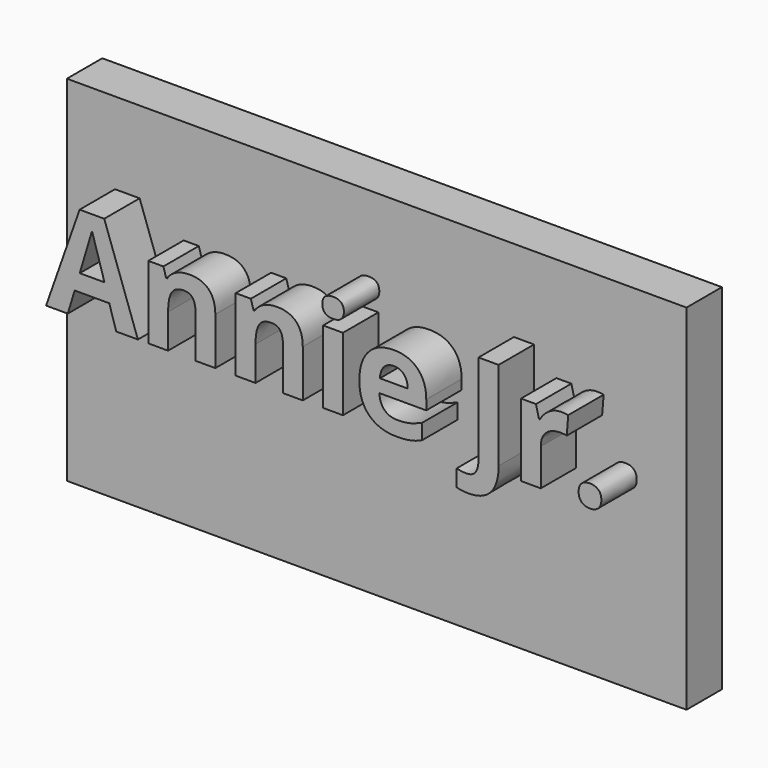
from build123d import *

# Parameters (mm, degrees)
F0_W         = 177.8
F0_H         = 101.6
F2_DEPTH     = 12.7
F3_TEXT_SIZE = 38.1786557328
F4_DEPTH     = 12.7


# Not quite as in the source:
# - Text() gives the source's letters only with a copy of the font that has no kerning and outlines rounded to 1/6400 em; it was checked with that copy


with BuildPart() as f2:
    # F0 (on Front) → F2 (new body)
    with BuildSketch(Plane.XZ):
        Rectangle(F0_W, F0_H)
    extrude(amount=F2_DEPTH)

    # F3 (on face) → F4 (join)
    with BuildSketch(Plane.XZ.offset(12.7)):
        with Locations((-84.7097373027, 0)):
            Text('Annie Jr.', F3_TEXT_SIZE, font='Open Sans', font_style=FontStyle.BOLD, text_align=(TextAlign.LEFT, TextAlign.BOTTOM))
    extrude(amount=F4_DEPTH)


solid = f2.part
